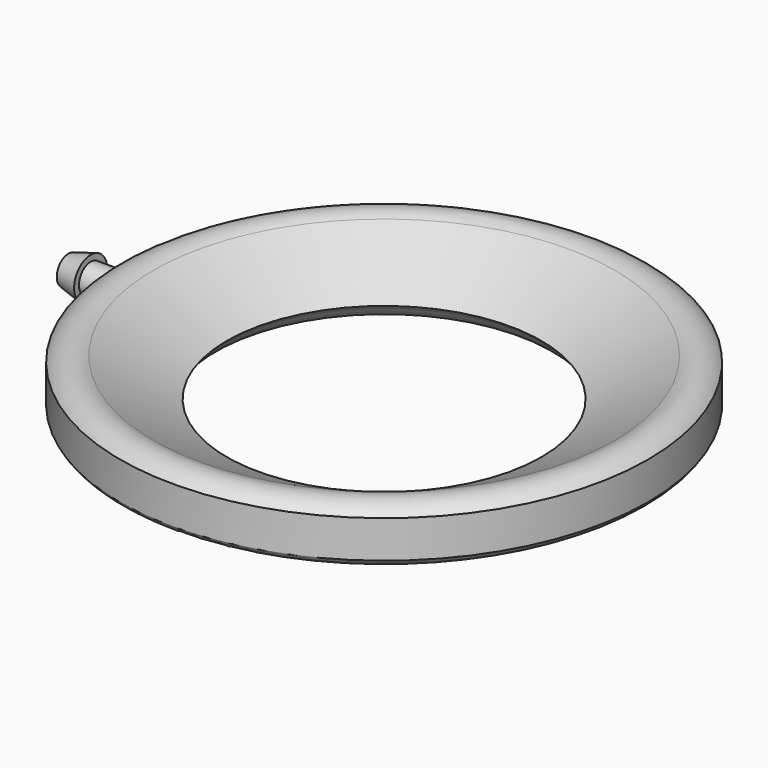
from build123d import *


# Not quite as in the source:
# - a feature names something its author has since deleted; it is built from what else it names


with BuildPart() as f1:
    # F0 (on Front) → F1 (revolve)
    with BuildSketch(Plane.XZ):
        with BuildLine():
            Line((22.3186584817, 4.9634656969), (15.2303930372, 1.2544910423))
            Line((15.2303930372, 1.2544910423), (15.488850391, 0.9470738952))
            Line((15.488850391, 0.9470738952), (15.5328564546, 0.894731726))
            Line((15.5328564546, 0.894731726), (15.8405525238, 1.0429841968))
            Line((15.8405525238, 1.0429841968), (22.4313864066, 4.2185444515))
            ThreePointArc((22.4313864066, 4.2185444515), (24.744105662, 3.4097946744), (23.9353558848, 1.097075419))
            Line((23.9353558848, 1.097075419), (16.3696151821, 0.4137007552))
            Line((16.3696151821, 0.4137007552), (15.9677918852, 0.3774061119))
            Line((15.9677918852, 0.3774061119), (16.2850916386, 0))
            Line((16.2850916386, 0), (24.2850916386, 0))
            ThreePointArc((24.2850916386, 0), (25.023915829, 0.2087553322), (25.5442474517, 0.7732860891))
            Line((25.5442474517, 0.7732860891), (25.5442474517, 4.3952541752))
            ThreePointArc((25.5442474517, 4.3952541752), (24.028202675, 5.2285828576), (22.3186584817, 4.9634656969))
        make_face()
        Polygon((15.8405525238, 1.0429841968), (15.5328564546, 0.894731726), (15.9677918852, 0.3774061119), (16.3696151821, 0.4137007552), align=None)
    revolve(axis=Axis((0, 0, 1.8443568842), (0, 0, 1)))

    # F2 (on Front) → F3 (revolve)
    with BuildSketch(Plane.XZ):
        Polygon((-25.3970567137, 3.7070766557), (-28.3970567137, 3.7070766557), (-28.3970567137, 4.2962685693), (-30.5454257131, 3.7070766557), (-30.5454257131, 3.2924627885), (-25.5454257131, 3.2924627885), align=None)
    revolve(axis=Axis((-26.2971473858, 0, 2.2924627885), (-1, 0, 0)))


solid = f1.part
